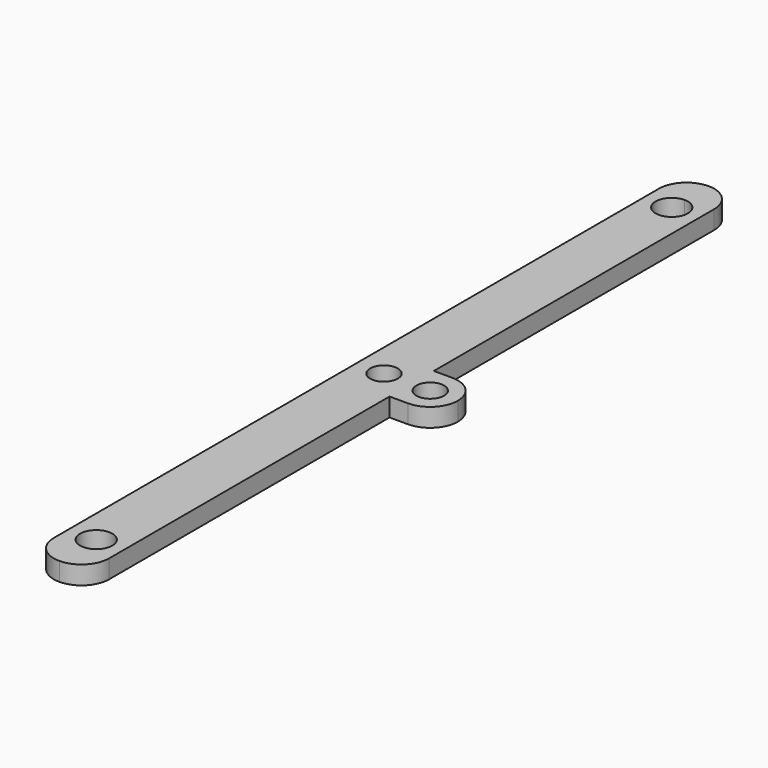
from build123d import *

# Parameters (mm, degrees)
F0_W     = 6
F0_H     = 88
F1_DEPTH = 2
F2_R     = 1.5
F3_DEPTH = 2
F5_DEPTH = 5
F6_R     = 1.5
F7_DEPTH = 2
F8_R     = 2.99999


# Not quite as in the source:
# - a fillet or chamfer is up to 0.001 mm smaller than in the source, because OpenCascade refuses the exact size


with BuildPart() as f1:
    # F0 (on Top) → F1 (new body)
    with BuildSketch(Plane.XY):
        Rectangle(F0_W, F0_H)
    extrude(amount=F1_DEPTH)

    # F2 (on face) → F3 (cut, through all)
    with BuildSketch(Plane.XY.offset(2)):
        Circle(F2_R)
        with BuildLine():
            ThreePointArc((0, 40.75), (-1.2374368671, 37.7625631329), (1.75, 39))
            ThreePointArc((1.75, 39), (1.2374368671, 40.2374368671), (0, 40.75))
        make_face()
        with BuildLine():
            ThreePointArc((0, -40.75), (1.2374368671, -40.2374368671), (1.75, -39))
            ThreePointArc((1.75, -39), (-1.2374368671, -37.7625631329), (0, -40.75))
        make_face()
    extrude(amount=-F3_DEPTH, mode=Mode.SUBTRACT)

    # F4 (on face) → F5 (join)
    with BuildSketch(Plane.YZ.offset(3)):
        Polygon((3, 2), (0, 2), (-3, 2), (-3, 0), (0, 0), (3, 0), align=None)
    extrude(amount=F5_DEPTH)

    # F6 (on face) → F7 (cut, through all)
    with BuildSketch(Plane.XY.offset(2)):
        with Locations((5.0139404441, 0)):
            Circle(F6_R)
    extrude(amount=-F7_DEPTH, mode=Mode.SUBTRACT)

    # F8 (radius 3 in the source; OpenCascade refuses exactly that, so slightly less here)
    f8_edges = [f1.edges().sort_by_distance(p)[0] for p in [
        (-3, -44, 1),
        (3, -44, 1),
        (3, 44, 1),
        (-3, 44, 1),
        (8, -3, 1),
        (8, 3, 1),
    ]]
    fillet(f8_edges, radius=F8_R)


solid = f1.part
